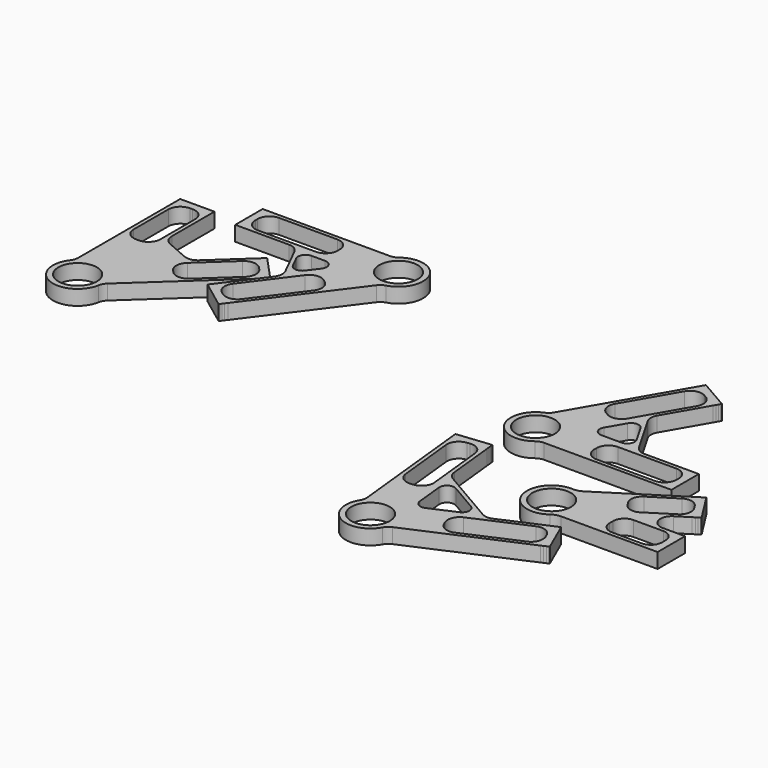
from build123d import *

# Parameters (mm, degrees)
F0_R     = 8.156575
F1_DEPTH = 6.35
F2_R     = 8.156575
F3_DEPTH = 6.35


# Not quite as in the source:
# - ends of sketch curves that miss each other by under 0.0002 mm in the source are joined


with BuildPart() as f1:
    # F0 (on Top) → F1 (new body)
    with BuildSketch(Plane.XY):
        with BuildLine():
            Line((-0.8965692, 213.555072), (-0.8965692, 216.730072))
            Line((-0.8965692, 216.730072), (-15.4355038, 216.730072))
            Line((-15.4355038, 216.730072), (-15.4355038, 213.555072))
            Line((-15.4355038, 213.555072), (-15.4355292, 162.6919022))
            ThreePointArc((-15.4355292, 162.6919022), (-15.704529087, 161.0607437428), (-16.4830401892, 159.6023338843))
            ThreePointArc((-16.4830401892, 159.6023338843), (-12.369087601, 143.6325476083), (2.1572627304, 151.4391959469))
            ThreePointArc((2.1572627304, 151.4391959469), (2.7011342813, 153.0003619517), (3.7174695963, 154.3042360534))
            Line((3.7174695963, 154.3042360534), (41.0975556, 188.7975904))
            Line((41.0975556, 188.7975904), (41.8955982, 189.5340126))
            Line((41.8955982, 189.5340126), (42.5974002, 190.1816364))
            Line((42.5974002, 190.1816364), (43.1183034, 190.6622806))
            Line((43.1183034, 190.6622806), (43.3954682, 190.9180332))
            Line((43.3954682, 190.9180332), (43.4309012, 190.9507484))
            Line((43.4309012, 190.9507484), (33.57118, 201.6356394))
            Line((33.57118, 201.6356394), (33.5357216, 201.6029496))
            Line((33.5357216, 201.6029496), (33.2585568, 201.3471716))
            Line((33.2585568, 201.3471716), (32.7376536, 200.8665274))
            Line((32.7376536, 200.8665274), (32.035877, 200.218929))
            Line((32.035877, 200.218929), (31.237809, 199.4825068))
            Line((31.237809, 199.4825068), (16.9377868, 186.2868004))
            ThreePointArc((16.9377868, 186.2868004), (14.3333605363, 185.010203827), (11.4548968936, 185.3668235744))
            Line((11.4548968936, 185.3668235744), (2.1456142, 189.443614))
            ThreePointArc((2.1456142, 189.443614), (-0.0685395805, 191.3171954099), (-0.8965692, 194.0969702))
            Line((-0.8965692, 194.0969702), (-0.8965692, 213.555072))
        make_face()
        with Locations((-8.1660492, 153.230072)):
            Circle(F0_R, mode=Mode.SUBTRACT)
        with BuildLine():
            ThreePointArc((-8.7680038, 184.980072), (-12.3601226682, 186.4679605713), (-13.8480292, 190.060072))
            Line((-13.8480292, 190.060072), (-13.8480292, 208.475072))
            ThreePointArc((-13.8480292, 208.475072), (-12.3601316484, 212.0671744484), (-8.7680292, 213.555072))
            Line((-8.7680292, 213.555072), (-7.5640692, 213.555072))
            ThreePointArc((-7.5640692, 213.555072), (-3.9719667516, 212.0671744484), (-2.4840692, 208.475072))
            Line((-2.4840692, 208.475072), (-2.4840692, 190.060072))
            ThreePointArc((-2.4840692, 190.060072), (-3.9719577713, 186.4679785318), (-7.5640438, 184.980072))
            Line((-7.5640438, 184.980072), (-8.7680038, 184.980072))
        make_face(mode=Mode.SUBTRACT)
        with BuildLine():
            ThreePointArc((14.7592561466, 175.2040455963), (13.4167148793, 178.8529662682), (15.0475713963, 182.3824628534))
            Line((15.0475713963, 182.3824628534), (28.5810198, 194.8707558))
            ThreePointArc((28.5810198, 194.8707558), (32.2299429884, 196.2133204917), (35.7594515125, 194.5824502851))
            Line((35.7594515125, 194.5824502851), (36.5759238, 193.6976314))
            ThreePointArc((36.5759238, 193.6976314), (37.9184627461, 190.0487250059), (36.2876066037, 186.5192377466))
            Line((36.2876066037, 186.5192377466), (22.7541582, 174.0309194))
            ThreePointArc((22.7541582, 174.0309194), (19.1052357318, 172.6883800793), (15.5757391466, 174.3192365963))
            Line((15.5757391466, 174.3192365963), (14.7592561466, 175.2040455963))
        make_face(mode=Mode.SUBTRACT)
    extrude(amount=F1_DEPTH)


with BuildPart() as f1b:
    # F0 (on Top) → F1, piece 2 (new body)
    with BuildSketch(Plane.XY):
        with BuildLine():
            Line((239.0060244, 155.4097476), (242.1810244, 155.4097476))
            Line((242.1810244, 155.4097476), (242.1810244, 169.9487076))
            Line((242.1810244, 169.9487076), (239.0060244, 169.9487076))
            Line((239.0060244, 169.9487076), (219.1597852, 169.9487076))
            ThreePointArc((219.1597852, 169.9487076), (216.6197856441, 170.6292982924), (214.7603766616, 172.4887067118))
            Line((214.7603766616, 172.4887067118), (205.2159726, 189.0201198))
            ThreePointArc((205.2159726, 189.0201198), (204.5353796, 191.5601198), (205.2159710616, 194.1001206882))
            Line((205.2159710616, 194.1001206882), (215.1390922, 211.2874616))
            Line((215.1390922, 211.2874616), (215.6820426, 212.2278966))
            Line((215.6820426, 212.2278966), (216.1595118, 213.0548952))
            Line((216.1595118, 213.0548952), (216.5138926, 213.6687116))
            Line((216.5138926, 213.6687116), (216.7024622, 213.9953302))
            Line((216.7024622, 213.9953302), (216.7265922, 214.0371132))
            Line((216.7265922, 214.0371132), (204.135482, 221.3065932))
            Line((204.135482, 221.3065932), (204.111352, 221.2648102))
            Line((204.111352, 221.2648102), (203.9227824, 220.9381916))
            Line((203.9227824, 220.9381916), (203.5684016, 220.3243752))
            Line((203.5684016, 220.3243752), (203.0909324, 219.4973766))
            Line((203.0909324, 219.4973766), (202.547982, 218.5569416))
            Line((202.547982, 218.5569416), (177.1163844, 174.50816))
            ThreePointArc((177.1163844, 174.50816), (176.0678390105, 173.2300287205), (174.6644137386, 172.3562636129))
            ThreePointArc((174.6644137386, 172.3562636129), (169.6072431076, 157.4404778153), (185.0532724434, 154.3622292759))
            ThreePointArc((185.0532724434, 154.3622292759), (186.5116888279, 155.1407452329), (188.1428546, 155.4097476))
            Line((188.1428546, 155.4097476), (239.0060244, 155.4097476))
        make_face()
        with Locations((178.6810244, 162.6792276)):
            Circle(F0_R, mode=Mode.SUBTRACT)
        with BuildLine():
            Line((239.0060244, 163.2812076), (239.0060244, 162.0772476))
            ThreePointArc((239.0060244, 162.0772476), (237.5181268484, 158.4851451516), (233.9260244, 156.9972476))
            Line((233.9260244, 156.9972476), (209.1610244, 156.9972476))
            ThreePointArc((209.1610244, 156.9972476), (205.5689219516, 158.4851451516), (204.0810244, 162.0772476))
            Line((204.0810244, 162.0772476), (204.0810244, 163.2812076))
            ThreePointArc((204.0810244, 163.2812076), (205.5689219516, 166.8733100484), (209.1610244, 168.3612076))
            Line((209.1610244, 168.3612076), (233.9260244, 168.3612076))
            ThreePointArc((233.9260244, 168.3612076), (237.5181268484, 166.8733100484), (239.0060244, 163.2812076))
        make_face(mode=Mode.SUBTRACT)
        with BuildLine():
            ThreePointArc((201.0005852572, 183.6213517299), (203.7502148, 185.2088498), (206.4998443428, 183.6213517299))
            Line((206.4998443428, 183.6213517299), (210.7268582, 176.2999776))
            ThreePointArc((210.7268582, 176.2999776), (210.7268346392, 173.1249730657), (207.9772066, 171.5374776))
            Line((207.9772066, 171.5374776), (199.523223, 171.5374776))
            ThreePointArc((199.523223, 171.5374776), (196.7735917859, 173.124978565), (196.7735934572, 176.2999795299))
            Line((196.7735934572, 176.2999795299), (201.0005852572, 183.6213517299))
        make_face(mode=Mode.SUBTRACT)
        with BuildLine():
            ThreePointArc((190.8597075619, 184.9772400631), (188.4927887836, 188.0618492178), (189.0002808616, 191.9166604882))
            Line((189.0002808616, 191.9166604882), (201.3827824, 213.3637846))
            ThreePointArc((201.3827824, 213.3637846), (204.4673896415, 215.730688063), (208.3221902882, 215.2231931384))
            Line((208.3221902882, 215.2231931384), (209.3648594, 214.6212116))
            ThreePointArc((209.3648594, 214.6212116), (211.731762863, 211.5366043585), (211.2242679384, 207.6818037118))
            Line((211.2242679384, 207.6818037118), (198.8417664, 186.2346796))
            ThreePointArc((198.8417664, 186.2346796), (195.7571591585, 183.867776137), (191.9023585118, 184.3752710616))
            Line((191.9023585118, 184.3752710616), (190.8597075619, 184.9772400631))
        make_face(mode=Mode.SUBTRACT)
    extrude(amount=F1_DEPTH)


with BuildPart() as f1c:
    # F0 (on Top) → F1, piece 3 (new body)
    with BuildSketch(Plane.XY):
        with BuildLine():
            Line((263.3302074, 117.6744916), (266.5052074, 117.6744916))
            Line((266.5052074, 117.6744916), (266.5052074, 132.2134516))
            Line((266.5052074, 132.2134516), (263.3302074, 132.2134516))
            Line((263.3302074, 132.2134516), (257.065653, 132.2134516))
            ThreePointArc((257.065653, 132.2134516), (252.4927189232, 135.6456583318), (254.5109681, 140.9952788213))
            Line((254.5109681, 140.9952788213), (259.7979564, 144.3556676))
            Line((259.7979564, 144.3556676), (260.7144138, 144.9381658))
            Line((260.7144138, 144.9381658), (261.5203558, 145.450433))
            Line((261.5203558, 145.450433), (262.1185258, 145.8306202))
            Line((262.1185258, 145.8306202), (262.4367878, 146.0329312))
            Line((262.4367878, 146.0329312), (262.477504, 146.0587884))
            Line((262.477504, 146.0587884), (254.6785864, 158.328995))
            Line((254.6785864, 158.328995), (254.6378702, 158.3031378))
            Line((254.6378702, 158.3031378), (254.3195828, 158.1008268))
            Line((254.3195828, 158.1008268), (253.7214128, 157.7206396))
            Line((253.7214128, 157.7206396), (252.9154962, 157.2083978))
            Line((252.9154962, 157.2083978), (251.9990388, 156.6258742))
            Line((251.9990388, 156.6258742), (220.1465498, 136.3804994))
            ThreePointArc((220.1465498, 136.3804994), (218.3255772444, 135.5906579393), (216.3497076456, 135.4016192761))
            ThreePointArc((216.3497076456, 135.4016192761), (205.6447499628, 122.0173348949), (221.8587852832, 116.4639075976))
            ThreePointArc((221.8587852832, 116.4639075976), (223.6277360061, 117.3642681975), (225.5882458, 117.6744916))
            Line((225.5882458, 117.6744916), (263.3302074, 117.6744916))
        make_face()
        with Locations((215.7052074, 124.9439716)):
            Circle(F0_R, mode=Mode.SUBTRACT)
        with BuildLine():
            ThreePointArc((241.1052074001, 125.8634262), (242.5001023744, 129.2310386651), (245.8677074, 130.6259516))
            Line((245.8677074, 130.6259516), (258.5677074, 130.6259516))
            ThreePointArc((258.5677074, 130.6259516), (261.9353034454, 129.2310476454), (263.3302074, 125.8634516))
            Line((263.3302074, 125.8634516), (263.3302074, 124.0244916))
            ThreePointArc((263.3302074, 124.0244916), (261.9353034454, 120.6568955546), (258.5677074, 119.2619916))
            Line((258.5677074, 119.2619916), (245.8677074, 119.2619916))
            ThreePointArc((245.8677074, 119.2619916), (242.5001113546, 120.6568955546), (241.1052074, 124.0244916))
            Line((241.1052074, 124.0244916), (241.1052074, 125.8634262))
        make_face(mode=Mode.SUBTRACT)
        with BuildLine():
            ThreePointArc((236.6483905787, 139.3449297), (236.0191915803, 142.9352835791), (238.1130509914, 145.9189533201))
            Line((238.1130509914, 145.9189533201), (248.8312524, 152.7314192))
            ThreePointArc((248.8312524, 152.7314192), (252.4215987668, 153.3606248691), (255.4052681299, 151.2667712012))
            Line((255.4052681299, 151.2667712012), (256.3917148, 149.7147882))
            ThreePointArc((256.3917148, 149.7147882), (257.0209204691, 146.1244418332), (254.9270668012, 143.1407724701))
            Line((254.9270668012, 143.1407724701), (244.2088588, 136.328277))
            ThreePointArc((244.2088588, 136.328277), (240.6185124332, 135.6990967309), (237.6348503787, 137.7929389))
            Line((237.6348503787, 137.7929389), (236.6483905787, 139.3449297))
        make_face(mode=Mode.SUBTRACT)
    extrude(amount=F1_DEPTH)


with BuildPart() as f1d:
    # F0 (on Top) → F1, piece 4 (new body)
    with BuildSketch(Plane.XY):
        with BuildLine():
            Line((236.1529694, 98.317431), (236.1971908, 98.336735))
            Line((236.1971908, 98.336735), (230.3765268, 111.6596954))
            Line((230.3765268, 111.6596954), (230.3323308, 111.6403914))
            Line((230.3323308, 111.6403914), (229.9867384, 111.4893884))
            Line((229.9867384, 111.4893884), (229.337235, 111.205645))
            Line((229.337235, 111.205645), (228.4621542, 110.8233242))
            Line((228.4621542, 110.8233242), (227.4670838, 110.3885778))
            Line((227.4670838, 110.3885778), (208.954751, 102.3007606))
            ThreePointArc((208.954751, 102.3007606), (206.6285666793, 101.8842933443), (204.365657306, 102.5653532694))
            Line((204.365657306, 102.5653532694), (180.630322, 116.3796504))
            ThreePointArc((180.630322, 116.3796504), (178.9203964228, 118.0108385129), (178.1334930107, 120.2391567249))
            Line((178.1334930107, 120.2391567249), (176.0217968, 140.3304534))
            Line((176.0217968, 140.3304534), (175.9082842, 141.4104106))
            Line((175.9082842, 141.4104106), (175.8084622, 142.3601166))
            Line((175.8084622, 142.3601166), (175.7343958, 143.0650174))
            Line((175.7343958, 143.0650174), (175.694975, 143.4400738))
            Line((175.694975, 143.4400738), (175.6899204, 143.4880544))
            Line((175.6899204, 143.4880544), (161.2306148, 141.9683216))
            Line((161.2306148, 141.9683216), (161.235644, 141.920341))
            Line((161.235644, 141.920341), (161.2750648, 141.5452846))
            Line((161.2750648, 141.5452846), (161.3491566, 140.8403838))
            Line((161.3491566, 140.8403838), (161.4489786, 139.8906778))
            Line((161.4489786, 139.8906778), (161.5624912, 138.8107206))
            Line((161.5624912, 138.8107206), (166.879143, 88.2261634))
            ThreePointArc((166.879143, 88.2261634), (166.782099458, 86.5758224297), (166.1602935813, 85.0440284587))
            ThreePointArc((166.1602935813, 85.0440284587), (169.827434574, 70.5205988147), (184.2668214513, 74.5057908114))
            ThreePointArc((184.2668214513, 74.5057908114), (185.2915791034, 75.8030625267), (186.6786165007, 76.7025996407))
            Line((186.6786165007, 76.7025996407), (233.2877478, 97.0656174))
            Line((233.2877478, 97.0656174), (234.2828182, 97.5003638))
            Line((234.2828182, 97.5003638), (235.157899, 97.8826846))
            Line((235.157899, 97.8826846), (235.8074024, 98.166428))
            Line((235.8074024, 98.166428), (236.1529694, 98.317431))
        make_face()
        with Locations((175.097821, 79.576041)):
            Circle(F0_R, mode=Mode.SUBTRACT)
        with BuildLine():
            ThreePointArc((180.9642750951, 108.5052179583), (182.3973102195, 111.5028925325), (185.7189840112, 111.5811596502))
            Line((185.7189840112, 111.5811596502), (197.6798688, 104.6197552))
            ThreePointArc((197.6798688, 104.6197552), (199.252528799, 101.6929350282), (197.3539122693, 98.9662447792))
            Line((197.3539122693, 98.9662447792), (186.6176608, 94.2757068))
            ThreePointArc((186.6176608, 94.2757068), (183.7494750811, 94.4410803235), (182.1889614951, 96.8532727583))
            Line((182.1889614951, 96.8532727583), (180.9642750951, 108.5052179583))
        make_face(mode=Mode.SUBTRACT)
        with BuildLine():
            Line((230.1363952, 104.2787348), (230.618411, 103.1754604))
            ThreePointArc((230.618411, 103.1754604), (230.6930360566, 99.288122794), (227.9970497809, 96.4865850882))
            Line((227.9970497809, 96.4865850882), (205.3033232, 86.5719376))
            ThreePointArc((205.3033232, 86.5719376), (201.4159903279, 86.4972852882), (198.6144478882, 89.1932734191))
            Line((198.6144478882, 89.1932734191), (198.1324206, 90.2965682))
            ThreePointArc((198.1324206, 90.2965682), (198.0577936882, 94.1839010721), (200.7537725007, 96.9854394407))
            Line((200.7537725007, 96.9854394407), (223.4475084, 106.900091))
            ThreePointArc((223.4475084, 106.900091), (227.3348558367, 106.9747221582), (230.1363952, 104.2787348))
        make_face(mode=Mode.SUBTRACT)
        with BuildLine():
            ThreePointArc((171.8441075931, 104.7739726478), (168.1161579662, 105.8782553291), (166.2609461703, 109.2951600473))
            Line((166.2609461703, 109.2951600473), (163.6722914, 133.9244718))
            ThreePointArc((163.6722914, 133.9244718), (164.7765547805, 137.6524358181), (168.1934674473, 139.5076574297))
            Line((168.1934674473, 139.5076574297), (169.3908474, 139.6335028))
            ThreePointArc((169.3908474, 139.6335028), (173.1187948021, 138.5292323063), (174.9740073522, 135.1123293931))
            Line((174.9740073522, 135.1123293931), (177.562637, 110.4829896))
            ThreePointArc((177.562637, 110.4829896), (176.4583736195, 106.7550509819), (173.0414860751, 104.8998320107))
            Line((173.0414860751, 104.8998320107), (171.8441075931, 104.7739726478))
        make_face(mode=Mode.SUBTRACT)
    extrude(amount=F1_DEPTH)


with BuildPart() as f3:
    # F2 (on face) → F3 (new body)
    with BuildSketch(Plane.XY.offset(6.35)):
        with BuildLine():
            Line((37.663755, 164.9738382), (37.6348498, 164.9352302))
            Line((37.6348498, 164.9352302), (49.272063, 156.2199568))
            Line((49.272063, 156.2199568), (49.3009936, 156.2585648))
            Line((49.3009936, 156.2585648), (49.5270536, 156.5604184))
            Line((49.5270536, 156.5604184), (49.9519448, 157.1277274))
            Line((49.9519448, 157.1277274), (50.5243592, 157.8920896))
            Line((50.5243592, 157.8920896), (51.1753104, 158.7612776))
            Line((51.1753104, 158.7612776), (81.6648608, 199.473058))
            ThreePointArc((81.6648608, 199.473058), (82.8579811117, 200.6174113413), (84.3553597217, 201.318074659))
            ThreePointArc((84.3553597217, 201.318074659), (90.8878005665, 216.0930464767), (75.1458261566, 219.7210967241))
            ThreePointArc((75.1458261566, 219.7210967241), (73.6874097721, 218.9425807671), (72.056244, 218.6735784))
            Line((72.056244, 218.6735784), (21.1930742, 218.6735784))
            Line((21.1930742, 218.6735784), (18.0180742, 218.6735784))
            Line((18.0180742, 218.6735784), (18.0180742, 204.1346184))
            Line((18.0180742, 204.1346184), (21.1930742, 204.1346184))
            Line((21.1930742, 204.1346184), (40.8338782, 204.1346184))
            ThreePointArc((40.8338782, 204.1346184), (43.5038385147, 203.3763902494), (45.3767755728, 201.3280482889))
            Line((45.3767755728, 201.3280482889), (51.7883902, 188.5159806))
            ThreePointArc((51.7883902, 188.5159806), (52.3051845557, 185.7889888335), (51.3116058038, 183.1973991461))
            Line((51.3116058038, 183.1973991461), (39.5380718, 167.476551))
            Line((39.5380718, 167.476551), (38.8871206, 166.607363))
            Line((38.8871206, 166.607363), (38.3147062, 165.8430262))
            Line((38.3147062, 165.8430262), (37.889815, 165.2756918))
            Line((37.889815, 165.2756918), (37.663755, 164.9738382))
        make_face()
        with BuildLine():
            ThreePointArc((56.1180742, 210.8021184), (54.6301766484, 207.2100159516), (51.0380742, 205.7221184))
            Line((51.0380742, 205.7221184), (26.2730742, 205.7221184))
            ThreePointArc((26.2730742, 205.7221184), (22.6809717516, 207.2100159516), (21.1930742, 210.8021184))
            Line((21.1930742, 210.8021184), (21.1930742, 212.0061038))
            ThreePointArc((21.1930742001, 212.0061038), (22.6809807318, 215.5981898287), (26.2730742, 217.0860784))
            Line((26.2730742, 217.0860784), (51.0380742, 217.0860784))
            ThreePointArc((51.0380742, 217.0860784), (54.6301766484, 215.5981808484), (56.1180742, 212.0060784))
            Line((56.1180742, 212.0060784), (56.1180742, 210.8021184))
        make_face(mode=Mode.SUBTRACT)
        with BuildLine():
            Line((45.8385164, 162.7580692), (44.8748658, 163.4797594))
            ThreePointArc((44.8748658, 163.4797594), (42.8915806166, 166.8239599624), (43.8538975232, 170.591059641))
            Line((43.8538975232, 170.591059641), (58.6990952, 190.413386))
            ThreePointArc((58.6990952, 190.413386), (62.0432957624, 192.3966711834), (65.810395441, 191.4343542768))
            Line((65.810395441, 191.4343542768), (66.77406, 190.7126488))
            ThreePointArc((66.77406, 190.7126488), (68.7573451834, 187.3684482376), (67.7950282768, 183.601348559))
            Line((67.7950282768, 183.601348559), (52.9498052, 163.7790222))
            ThreePointArc((52.9498052, 163.7790222), (49.6056124398, 161.7957344901), (45.8385164, 162.7580692))
        make_face(mode=Mode.SUBTRACT)
        with BuildLine():
            ThreePointArc((56.5426427139, 192.8326287728), (53.7178389945, 191.573536572), (51.1620060822, 193.3149576434))
            Line((51.1620060822, 193.3149576434), (48.8424728, 197.9499724))
            ThreePointArc((48.8424728, 197.9499724), (48.9806834717, 201.0395808443), (51.6817864, 202.5458484))
            Line((51.6817864, 202.5458484), (57.4725038, 202.5458484))
            ThreePointArc((57.4725038, 202.5458484), (60.311811288, 200.7917488148), (60.0138412408, 197.4676329598))
            Line((60.0138412408, 197.4676329598), (56.5426427139, 192.8326287728))
        make_face(mode=Mode.SUBTRACT)
        with Locations((81.5180742, 211.4040984)):
            Circle(F2_R, mode=Mode.SUBTRACT)
    extrude(amount=F3_DEPTH)


solid = Compound([f1.part, f1b.part, f1c.part, f1d.part, f3.part])
